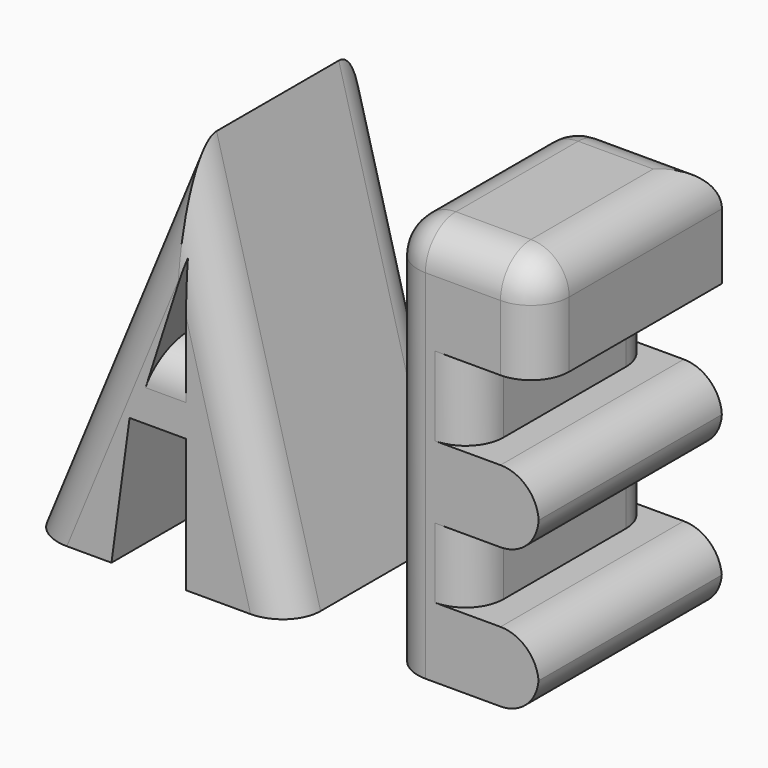
from build123d import *

# Parameters (mm, degrees)
F1_DEPTH       = 30
F2_T1_DEPTH    = 80.0888645747
F2_T3_DEPTH    = 77.7106724757
F2_2_T1_DEPTH  = 46.8092103302
F2_2_T3_DEPTH  = 14.835527055
F2_2_T5_DEPTH  = 9.835527055
F2_2_T7_DEPTH  = 20
F2_2_T9_DEPTH  = 8.6184208095
F2_2_T11_DEPTH = 25
F2_2_T13_DEPTH = 30
F2_2_S17_W     = 5.1
F2_2_S17_H     = 5.1
F2_2_T18_DEPTH = 5.1
F2_2_S23_W     = 5.1
F2_2_S23_H     = 5.1
F2_2_T24_DEPTH = 5.1
F2_2_S29_W     = 5.1
F2_2_S29_H     = 5.1
F2_2_T30_DEPTH = 5.1
F2_2_T37_DEPTH = 37.5
F2_2_T41_DEPTH = 27.335527055
F3_R           = 5
F3_2_R         = 5


# Not quite as in the source:
# - a fillet or chamfer that OpenCascade refuses, or shapes differently, is made with other operations: its cross-section is extruded or revolved along the edge and cut away or added


with BuildPart() as f1:
    # F0 (on Front) → F1 (new body)
    with BuildSketch(Plane.XZ):
        Polygon((-37.5986844301, 50.9210526943), (-58.6184225976, 0), (-47.3684221506, 0), (-45.0000017881, 17.4671057612), (-37.5986844301, 17.4671057612), (-37.5986844301, 0), (-23.9802636206, 0), align=None)
        Polygon((-37.5986844301, 26.6447365284), (-41.2993431091, 26.6447365284), (-37.5986844301, 38.1907895207), align=None, mode=Mode.SUBTRACT)
    extrude(amount=F1_DEPTH)

    # F2: fillet of radius 5 on 4 edges, made by hand

    # F2_s2 → F2_t1 (cut)
    with BuildSketch(Plane(origin=(17.2550791502, 0, 41.8010342303), x_dir=(0, 1, 0), z_dir=(-0.3815605627, 0, -0.9243438413))):
        with BuildLine():
            ThreePointArc((-25, -54.1835779154), (-28.5355339059, -52.7191118213), (-30, -49.1835779154))
            Line((-30, -49.1835779154), (-30, -54.1835779154))
            Line((-30, -54.1835779154), (-25, -54.1835779154))
        make_face()
        with BuildLine():
            ThreePointArc((-5, -54.1835779154), (-1.4644660941, -52.7191118213), (0, -49.1835779154))
            Line((0, -49.1835779154), (0, -54.1835779154))
            Line((0, -54.1835779154), (-5, -54.1835779154))
        make_face()
    extrude(amount=F2_T1_DEPTH, mode=Mode.SUBTRACT)

    # F2_s4 → F2_t3 (cut)
    with BuildSketch(Plane(origin=(1.6288202397, 0, -6.0903714472), x_dir=(0, 1, 0), z_dir=(-0.2583617353, 0, 0.9660482461))):
        with BuildLine():
            ThreePointArc((-25, 23.166091611), (-28.5355339059, 24.6305577051), (-30, 28.166091611))
            Line((-30, 28.166091611), (-30, 23.166091611))
            Line((-30, 23.166091611), (-25, 23.166091611))
        make_face()
        with BuildLine():
            ThreePointArc((-5, 23.166091611), (-1.4644660941, 24.6305577051), (0, 28.166091611))
            Line((0, 28.166091611), (0, 23.166091611))
            Line((0, 23.166091611), (-5, 23.166091611))
        make_face()
    extrude(amount=F2_T3_DEPTH, mode=Mode.SUBTRACT)

    # F3
    f3_edges = [f1.edges().sort_by_distance(p)[0] for p in [
        (-39.449014, -30, 26.644737),
    ]]
    fillet(f3_edges, radius=F3_R)


with BuildPart() as f1b:
    # F0 (on Front) → F1, piece 2 (new body)
    with BuildSketch(Plane.XZ):
        Polygon((-11.250000447, 51.8092103302), (-11.250000447, 0), (8.5855266079, 0), (8.5855266079, 9.1776316985), (0, 9.1776316985), (0, 18.3552633971), (8.5855266079, 18.3552633971), (8.5855266079, 27.8289485723), (0, 27.8289485723), (0, 38.1907895207), (8.5855266079, 38.1907895207), (8.5855266079, 51.8092103302), align=None)
    extrude(amount=F1_DEPTH)

    # F2#2: fillet of radius 5 on 11 edges, made by hand

    # F2_2_s2 → F2_2_t1 (cut)
    with BuildSketch(Plane.XY):
        with BuildLine():
            ThreePointArc((-11.250000447, -5), (-9.785534353, -1.4644660941), (-6.250000447, 0))
            Line((-6.250000447, 0), (-6.250000447, 0.1))
            Line((-6.250000447, 0.1), (-11.350000447, 0.1))
            Line((-11.350000447, 0.1), (-11.350000447, -5))
            Line((-11.350000447, -5), (-11.250000447, -5))
        make_face()
        with BuildLine():
            ThreePointArc((-11.250000447, -25), (-9.785534353, -28.5355339059), (-6.250000447, -30))
            Line((-6.250000447, -30), (-6.250000447, -30.1))
            Line((-6.250000447, -30.1), (-11.350000447, -30.1))
            Line((-11.350000447, -30.1), (-11.350000447, -25))
            Line((-11.350000447, -25), (-11.250000447, -25))
        make_face()
    extrude(amount=F2_2_T1_DEPTH, mode=Mode.SUBTRACT)

    # F2_2_s4 → F2_2_t3 (cut)
    with BuildSketch(Plane.YZ.offset(-6.250000447)):
        with BuildLine():
            ThreePointArc((-5, 51.8092103302), (-1.4644660941, 50.3447442362), (0, 46.8092103302))
            Line((0, 46.8092103302), (0.1, 46.8092103302))
            Line((0.1, 46.8092103302), (0.1, 51.9092103302))
            Line((0.1, 51.9092103302), (-5, 51.9092103302))
            Line((-5, 51.9092103302), (-5, 51.8092103302))
        make_face()
    extrude(amount=F2_2_T3_DEPTH, mode=Mode.SUBTRACT)

    # F2_2_s6 → F2_2_t5 (cut)
    with BuildSketch(Plane.YZ.offset(-6.250000447)):
        with BuildLine():
            ThreePointArc((-25, 51.8092103302), (-28.5355339059, 50.3447442362), (-30, 46.8092103302))
            Line((-30, 46.8092103302), (-30.1, 46.8092103302))
            Line((-30.1, 46.8092103302), (-30.1, 51.9092103302))
            Line((-30.1, 51.9092103302), (-25, 51.9092103302))
            Line((-25, 51.9092103302), (-25, 51.8092103302))
        make_face()
    extrude(amount=F2_2_T5_DEPTH, mode=Mode.SUBTRACT)

    # F2_2_s8 → F2_2_t7 (cut)
    with BuildSketch(Plane.XZ.offset(5)):
        with BuildLine():
            ThreePointArc((-11.250000447, 46.8092103302), (-9.785534353, 50.3447442362), (-6.250000447, 51.8092103302))
            Line((-6.250000447, 51.8092103302), (-6.250000447, 51.9092103302))
            Line((-6.250000447, 51.9092103302), (-11.350000447, 51.9092103302))
            Line((-11.350000447, 51.9092103302), (-11.350000447, 46.8092103302))
            Line((-11.350000447, 46.8092103302), (-11.250000447, 46.8092103302))
        make_face()
    extrude(amount=F2_2_T7_DEPTH, mode=Mode.SUBTRACT)

    # F2_2_s10 → F2_2_t9 (cut)
    with BuildSketch(Plane.XY.offset(38.1907895207)):
        with BuildLine():
            ThreePointArc((8.5855266079, -25), (7.1210605139, -28.5355339059), (3.5855266079, -30))
            Line((3.5855266079, -30), (3.5855266079, -30.1))
            Line((3.5855266079, -30.1), (8.6855266079, -30.1))
            Line((8.6855266079, -30.1), (8.6855266079, -25))
            Line((8.6855266079, -25), (8.5855266079, -25))
        make_face()
    extrude(amount=F2_2_T9_DEPTH, mode=Mode.SUBTRACT)

    # F2_2_s12 → F2_2_t11 (cut)
    with BuildSketch(Plane.XZ):
        with BuildLine():
            ThreePointArc((8.5855266079, 46.8092103302), (7.1210605139, 50.3447442362), (3.5855266079, 51.8092103302))
            Line((3.5855266079, 51.8092103302), (3.5855266079, 51.9092103302))
            Line((3.5855266079, 51.9092103302), (8.6855266079, 51.9092103302))
            Line((8.6855266079, 51.9092103302), (8.6855266079, 46.8092103302))
            Line((8.6855266079, 46.8092103302), (8.5855266079, 46.8092103302))
        make_face()
    extrude(amount=F2_2_T11_DEPTH, mode=Mode.SUBTRACT)

    # F2_2_s14 → F2_2_t13 (cut)
    with BuildSketch(Plane.XZ):
        with BuildLine():
            ThreePointArc((8.5855266079, 22.8289485723), (7.1210605139, 26.3644824782), (3.5855266079, 27.8289485723))
            Line((3.5855266079, 27.8289485723), (3.5855266079, 27.9289485723))
            Line((3.5855266079, 27.9289485723), (8.6855266079, 27.9289485723))
            Line((8.6855266079, 27.9289485723), (8.6855266079, 22.8289485723))
            Line((8.6855266079, 22.8289485723), (8.5855266079, 22.8289485723))
        make_face()
        with BuildLine():
            ThreePointArc((3.5855266079, 18.3552633971), (7.1210605139, 19.8197294912), (8.5855266079, 23.3552633971))
            Line((8.5855266079, 23.3552633971), (8.6855266079, 23.3552633971))
            Line((8.6855266079, 23.3552633971), (8.6855266079, 18.2552633971))
            Line((8.6855266079, 18.2552633971), (3.5855266079, 18.2552633971))
            Line((3.5855266079, 18.2552633971), (3.5855266079, 18.3552633971))
        make_face()
        with BuildLine():
            ThreePointArc((8.5855266079, 4.1776316985), (7.1210605139, 7.7131656045), (3.5855266079, 9.1776316985))
            Line((3.5855266079, 9.1776316985), (3.5855266079, 9.2776316985))
            Line((3.5855266079, 9.2776316985), (8.6855266079, 9.2776316985))
            Line((8.6855266079, 9.2776316985), (8.6855266079, 4.1776316985))
            Line((8.6855266079, 4.1776316985), (8.5855266079, 4.1776316985))
        make_face()
        with BuildLine():
            ThreePointArc((3.5855266079, 0), (7.1210605139, 1.4644660941), (8.5855266079, 5))
            Line((8.5855266079, 5), (8.6855266079, 5))
            Line((8.6855266079, 5), (8.6855266079, -0.1))
            Line((8.6855266079, -0.1), (3.5855266079, -0.1))
            Line((3.5855266079, -0.1), (3.5855266079, 0))
        make_face()
    extrude(amount=F2_2_T13_DEPTH, mode=Mode.SUBTRACT)


with BuildPart() as f2_2_tool16:
    # F2_2_s17 → F2_2_t18 (new body)
    with BuildSketch(Plane.YZ.offset(-6.250000447)):
        with Locations((-2.45, 49.3592103302)):
            Rectangle(F2_2_S17_W, F2_2_S17_H)
    extrude(amount=-F2_2_T18_DEPTH)

    # F2_2_s19 → F2_2_t20 (revolve, cut)
    with BuildSketch(Plane(origin=(-6.250000447, -5, 46.8092103302), x_dir=(0, -0.7071067812, -0.7071067812), z_dir=(0, 0.7071067812, -0.7071067812))):
        with BuildLine():
            ThreePointArc((0, -5), (5, 0), (0, 5))
            Line((0, 5), (0, -5))
        make_face()
    revolve(axis=Axis((-6.250000447, -5, 46.8092103302), (-1, 0, 0)), mode=Mode.SUBTRACT)


with BuildPart() as f1b_1:
    add(f1b.part)

    # F2_2_t15: cut F2_2_tool16
    add(f2_2_tool16.part, mode=Mode.SUBTRACT)


with BuildPart() as f2_2_tool22:
    # F2_2_s23 → F2_2_t24 (new body)
    with BuildSketch(Plane.YZ.offset(3.5855266079)):
        with Locations((-27.55, 49.3592103302)):
            Rectangle(F2_2_S23_W, F2_2_S23_H)
    extrude(amount=F2_2_T24_DEPTH)

    # F2_2_s25 → F2_2_t26 (revolve, cut)
    with BuildSketch(Plane(origin=(3.5855266079, -25, 46.8092103302), x_dir=(0, 0.7071067812, -0.7071067812), z_dir=(0, -0.7071067812, -0.7071067812))):
        with BuildLine():
            ThreePointArc((0, -5), (5, 0), (0, 5))
            Line((0, 5), (0, -5))
        make_face()
    revolve(axis=Axis((3.5855266079, -25, 46.8092103302), (1, 0, 0)), mode=Mode.SUBTRACT)


with BuildPart() as f1b_2:
    add(f1b_1.part)

    # F2_2_t21: cut F2_2_tool22
    add(f2_2_tool22.part, mode=Mode.SUBTRACT)


with BuildPart() as f2_2_tool28:
    # F2_2_s29 → F2_2_t30 (new body)
    with BuildSketch(Plane.YZ.offset(-6.250000447)):
        with Locations((-27.55, 49.3592103302)):
            Rectangle(F2_2_S29_W, F2_2_S29_H)
    extrude(amount=-F2_2_T30_DEPTH)

    # F2_2_s31 → F2_2_t32 (revolve, cut)
    with BuildSketch(Plane(origin=(-6.250000447, -25, 46.8092103302), x_dir=(0, 0.7071067812, -0.7071067812), z_dir=(0, 0.7071067812, 0.7071067812))):
        with BuildLine():
            ThreePointArc((0, -5), (5, 0), (0, 5))
            Line((0, 5), (0, -5))
        make_face()
    revolve(axis=Axis((-6.250000447, -25, 46.8092103302), (-1, 0, 0)), mode=Mode.SUBTRACT)


with BuildPart() as f1b_3:
    add(f1b_2.part)

    # F2_2_t27: cut F2_2_tool28
    add(f2_2_tool28.part, mode=Mode.SUBTRACT)


with BuildPart() as f2_2_tool35:
    # F2_2_s36 → F2_2_t37 (new body)
    with BuildSketch(Plane.XZ.offset(-12.5)):
        with BuildLine():
            ThreePointArc((8.5855266079, 46.8092103302), (7.1210605139, 50.3447442362), (3.5855266079, 51.8092103302))
            Line((3.5855266079, 51.8092103302), (3.5855266079, 51.9092103302))
            Line((3.5855266079, 51.9092103302), (8.6855266079, 51.9092103302))
            Line((8.6855266079, 51.9092103302), (8.6855266079, 46.8092103302))
            Line((8.6855266079, 46.8092103302), (8.5855266079, 46.8092103302))
        make_face()
    extrude(amount=F2_2_T37_DEPTH)

    split(bisect_by=Plane.XZ, keep=Keep.BOTTOM)


with BuildPart() as f2_2_tool39:
    # F2_2_s40 → F2_2_t41 (new body)
    with BuildSketch(Plane.YZ.offset(21.0855266079)):
        with BuildLine():
            ThreePointArc((-5, 51.8092103302), (-1.4644660941, 50.3447442362), (0, 46.8092103302))
            Line((0, 46.8092103302), (0.1, 46.8092103302))
            Line((0.1, 46.8092103302), (0.1, 51.9092103302))
            Line((0.1, 51.9092103302), (-5, 51.9092103302))
            Line((-5, 51.9092103302), (-5, 51.8092103302))
        make_face()
    extrude(amount=-F2_2_T41_DEPTH)

    split(bisect_by=Plane.YZ.offset(8.5855266079), keep=Keep.TOP)


with BuildPart() as f2_2_tool35_1:
    add(f2_2_tool35.part)

    # F2_2_t43: intersect F2_2_tool39
    add(f2_2_tool39.part, mode=Mode.INTERSECT)


with BuildPart() as f1b_4:
    add(f1b_3.part)

    # F2_2_t33: cut F2_2_tool35
    add(f2_2_tool35_1.part, mode=Mode.SUBTRACT)

    # F3#2
    f3_2_edges = [f1b_4.edges().sort_by_distance(p)[0] for p in [
        (0, 0, 33.009869),
        (0, 0, 13.766448),
        (0, -30, 13.766448),
        (0, -30, 33.009869),
    ]]
    fillet(f3_2_edges, radius=F3_2_R)


solid = Compound([f1.part, f1b_4.part])
